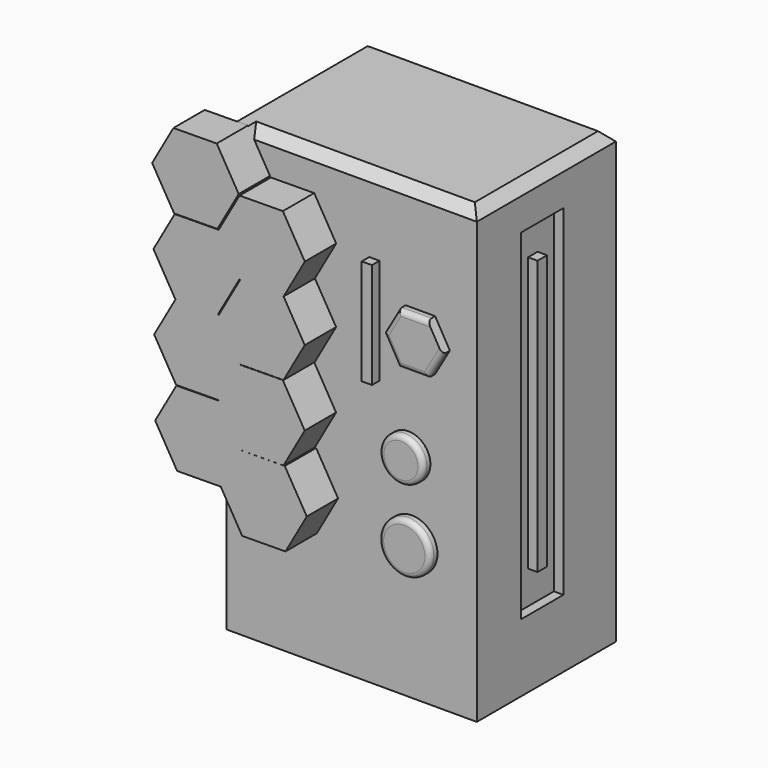
from build123d import *

# Parameters (mm, degrees)
F0_W      = 127.7551352978
F0_H      = 88.7857824564
F1_DEPTH  = 230
F4_DEPTH  = 20
F5_DEPTH  = 19.9898
F6_W      = 26.9565298222
F6_H      = 173.913128674
F6_W_2    = 6.0869585723
F6_H_2    = 140.0000751019
F7_DEPTH  = 4.826
F8_SIZE   = 5.08
F9_R      = 13.0796675924
F9_R_2    = 11.2186028003
F9_W      = 5.2173919976
F9_H      = 53.9130866528
F10_DEPTH = 4.826
F11_R     = 2.54


with BuildPart() as f1:
    # F0 (on Top) → F1 (new body)
    with BuildSketch(Plane.XY):
        Rectangle(F0_W, F0_H)
    extrude(amount=F1_DEPTH)

    # F3 (on face) → F4 (join)
    with BuildSketch(Plane.XZ.offset(44.3928912282)):
        Polygon((-41.2921301063, 173.0379974811), (-41.085819379, 172.688162985), (-41.1297441764, 172.6104329043), (-40.9572269026, 172.3179008855), (-18.8467815635, 172.5222300093), (-18.8301746286, 172.5516179285), (-19.2372092384, 173.2418134869), align=None)
        Polygon((-40.9572269026, 172.3179008855), (-41.1297441764, 172.6104329043), (-51.9640878366, 153.4377910705), (-40.9382216824, 134.7415827759), (-18.8833008145, 134.9453987817), (-8.0050323569, 154.1957706962), (-18.8301746286, 172.5516179285), (-18.8467815635, 172.5222300093), align=None)
        Polygon((-41.3476545775, 173.0374843632), (-41.2921301063, 173.0379974811), (-52.1454789867, 191.4416737569), (-52.1894037841, 191.3639436762), (-41.3642615124, 173.008096444), align=None)
        Polygon((-52.1454789867, 191.4416737569), (-41.2921301063, 173.0379974811), (-19.2372092384, 173.2418134869), (-18.8301746286, 172.5516179285), (-7.968513106, 191.7726019238), (-19.2006899874, 210.8186447145), (-41.3111353265, 210.6143155907), align=None)
        Polygon((-40.9382216824, 134.7415827759), (-51.9640878366, 153.4377910705), (-52.0196123078, 153.4372779525), (-40.9937461536, 134.7410696579), align=None)
        Polygon((-52.225923035, 153.7871124486), (-41.3642615124, 173.008096444), (-52.1894037841, 191.3639436762), (-52.1454789867, 191.4416737569), (-52.3179962605, 191.7342057757), (-74.4284415995, 191.5298766519), (-85.3067100571, 172.2795047374), (-74.0745331757, 153.2334619467), (-52.0196123078, 153.4372779525), align=None)
        Polygon((-40.9937461536, 134.7410696579), (-52.0196123078, 153.4372779525), (-74.0745331757, 153.2334619467), (-84.9528016333, 133.9830900322), (-73.7206247518, 114.9370472415), (-52.1037964015, 115.1368147056), (-52.2374327127, 115.3634175206), (-41.3591642551, 134.6137894351), (-40.8655472663, 134.6183510948), (-40.9382216824, 134.7415827759), align=None)
        Polygon((-19.248718916, 134.8181185589), (-40.8655472663, 134.6183510948), (-40.7319109552, 134.3917482798), (-51.6101794127, 115.1413763653), (-52.1037964015, 115.1368147056), (-51.9623043786, 114.8968912116), (-51.4474166697, 114.9016494402), (-40.4903681222, 96.3221329585), (-18.8948104921, 96.5217038537), (-8.0165420346, 115.7720757682), align=None)
        Polygon((-40.7319109552, 134.3917482798), (-40.8655472663, 134.6183510948), (-41.3591642551, 134.6137894351), (-52.2374327127, 115.3634175206), (-52.1037964015, 115.1368147056), (-51.6101794127, 115.1413763653), align=None)
        Polygon((-41.0052558312, 96.3173747299), (-51.9623043786, 114.8968912116), (-73.5578620087, 114.6973203164), (-84.4361304663, 95.4469484019), (-73.2039535849, 76.4009056112), (-51.0935082458, 76.605234735), (-51.0213053835, 76.7330061684), (-51.2069400891, 77.0477809963), (-40.4008744938, 96.1703814775), (-40.4903681222, 96.3221329585), align=None)
        Polygon((-51.4474166697, 114.9016494402), (-51.9623043786, 114.8968912116), (-41.0052558312, 96.3173747299), (-40.4903681222, 96.3221329585), align=None)
        Polygon((-40.3286716315, 96.2981529109), (-40.4008744938, 96.1703814775), (-40.2152397882, 95.8556066495), (-51.0213053835, 76.7330061684), (-39.9747632076, 58.0017382056), (-17.8643178685, 58.2060673294), (-6.986049411, 77.4564392439), (-18.2182262924, 96.5024820346), align=None)
        Polygon((-40.2152397882, 95.8556066495), (-40.4008744938, 96.1703814775), (-51.2069400891, 77.0477809963), (-51.0213053835, 76.7330061684), align=None)
    extrude(amount=F4_DEPTH)

    # F2 (on face) → F5 (join)
    with BuildSketch(Plane.XZ.offset(44.3928912282)):
        Polygon((-52.6453907674, 191.9314519259), (-41.7671223098, 211.1818238404), (-52.9992991913, 230.2278666311), (-75.1097445304, 230.0235375074), (-85.9880129879, 210.7731655929), (-74.7558361065, 191.7271228021), align=None)
    extrude(amount=F5_DEPTH)

    # F6 (on face) → F7 (cut)
    with BuildSketch(Plane.YZ.offset(63.8775676489)):
        with Locations((-2.6086920407, 121.6356754303)):
            Rectangle(F6_W, F6_H)
        with Locations((-2.6086920407, 121.6356754303)):
            Rectangle(F6_W_2, F6_H_2, mode=Mode.SUBTRACT)
    extrude(amount=-F7_DEPTH, mode=Mode.SUBTRACT)

    # F8
    f8_edges = [f1.edges().sort_by_distance(p)[0] for p in [
        (5.506325, -44.392891, 230),
        (63.877568, 0, 230),
        (0, 44.392891, 230),
        (-63.877568, 0, 230),
    ]]
    chamfer(f8_edges, length=F8_SIZE)

    # F9 (on face) → F10 (join)
    with BuildSketch(Plane.XZ.offset(44.3928912282)):
        with Locations((30.683927238, 69.0269544721)):
            Circle(F9_R)
        with Locations((28.9447959512, 108.1574112177)):
            Circle(F9_R_2)
        with Locations((11.5534868091, 164.2443984747)):
            Rectangle(F9_W, F9_H)
        Polygon((27.5010903101, 149.4617760181), (42.562418737, 149.4617760181), (50.0930829504, 162.5052690506), (42.562418737, 175.5487620831), (27.5010903101, 175.5487620831), (19.9704260966, 162.5052690506), align=None)
    extrude(amount=F10_DEPTH)

    # F11
    f11_edges = [f1.edges().sort_by_distance(p)[0] for p in [
        (35.031755, -49.218891, 175.548762),
        (46.327751, -49.218891, 155.983523),
        (35.031755, -49.218891, 149.461776),
        (23.735758, -49.218891, 155.983523),
        (23.735758, -49.218891, 169.027016),
        (17.726193, -49.218891, 108.157411),
        (17.60426, -49.218891, 69.026954),
    ]]
    fillet(f11_edges, radius=F11_R)


solid = f1.part
